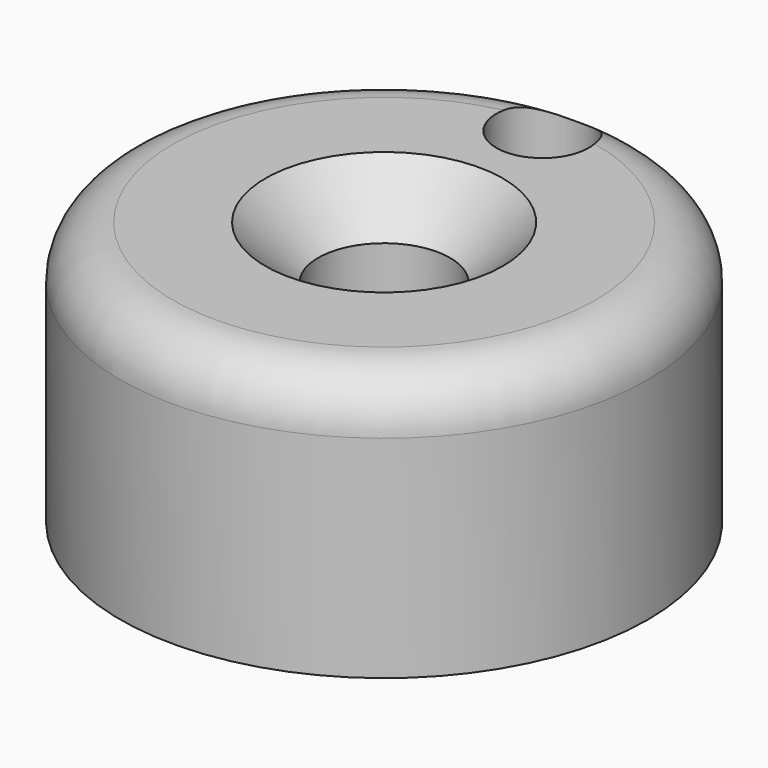
from build123d import *

# Parameters (mm, degrees)
F0_R     = 25.4
F0_R_2   = 6.35
F0_R_3   = 4.445
F1_DEPTH = 25.4
F3_SIZE  = 5.08


# Not quite as in the source:
# - a fillet or chamfer that OpenCascade refuses, or shapes differently, is made with other operations: its cross-section is extruded or revolved along the edge and cut away or added


with BuildPart() as f1:
    # F0 (on Top) → F1 (new body)
    with BuildSketch(Plane.XY):
        Circle(F0_R)
        Circle(F0_R_2, mode=Mode.SUBTRACT)
        with Locations((0, 19.05)):
            Circle(F0_R_3, mode=Mode.SUBTRACT)
    extrude(amount=F1_DEPTH)

    # F2: fillet of radius 5.08 on 1 edges, made by hand

    # F2_s1 → F2_t2 (revolve, cut)
    with BuildSketch(Plane.XZ):
        with BuildLine():
            ThreePointArc((25.4, 20.32), (23.9121024484, 23.9121024484), (20.32, 25.4))
            Line((20.32, 25.4), (25.4, 25.4))
            Line((25.4, 25.4), (25.4, 20.32))
        make_face()
    revolve(axis=Axis((0, 0, 25.4), (0, 0, 1)), mode=Mode.SUBTRACT)

    # F3
    f3_edges = [f1.edges().sort_by_distance(p)[0] for p in [
        (-6.35, 0, 25.4),
    ]]
    chamfer(f3_edges, length=F3_SIZE)


solid = f1.part
